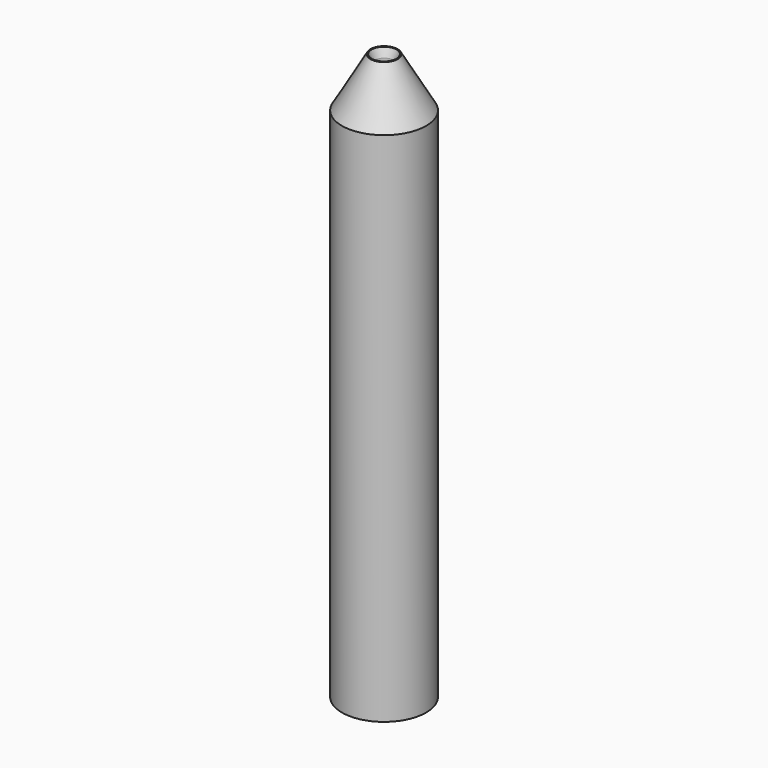
from build123d import *

# Parameters (mm, degrees)
F0_R      = 3.5
F1_DEPTH  = 25
F2_DEPTH  = 47
F3_R      = 1.65
F4_DEPTH  = 38
F5_R      = 1.13
F6_DEPTH  = 100
F6_TAPER  = -30
F8_R      = 1.03
F9_DEPTH  = 2
F9_TAPER  = 22.5
F10_R     = 0.75
F11_DEPTH = 5


# Not quite as in the source:
# - a feature names something its author has since deleted; it is built from what else it names


with BuildPart() as f1:
    # F0 (on Top) → F1 (new body)
    with BuildSketch(Plane.XY):
        Circle(F0_R)
    extrude(amount=F1_DEPTH)


with BuildPart() as f2:
    # F0 (on Top) → F2 (new body)
    with BuildSketch(Plane.XY):
        Circle(F0_R)
    extrude(amount=F2_DEPTH)


with BuildPart() as f4_tool:
    # F3 (on face) → F4 (new body)
    with BuildSketch(Plane(origin=(0, 0, 0), x_dir=(1, 0, 0), z_dir=(0, 0, -1))):
        Circle(F3_R)
    extrude(amount=-F4_DEPTH)


with BuildPart() as f1_1:
    add(f1.part)

    # F4: cut by f4_tool
    add(f4_tool.part, mode=Mode.SUBTRACT)


with BuildPart() as f2_1:
    add(f2.part)

    # F4: cut by f4_tool
    add(f4_tool.part, mode=Mode.SUBTRACT)


with BuildPart() as f6_tool:
    # F5 (on face) → F6 (new body)
    with BuildSketch(Plane.XY.offset(47)):
        Circle(F5_R)
    extrude(amount=-F6_DEPTH, taper=F6_TAPER)


with BuildPart() as f1_2:
    add(f1_1.part)

    # F6: intersect by f6_tool
    add(f6_tool.part, mode=Mode.INTERSECT)


with BuildPart() as f2_2:
    add(f2_1.part)

    # F6: intersect by f6_tool
    add(f6_tool.part, mode=Mode.INTERSECT)

    # F8 (on face) → F9 (cut)
    with BuildSketch(Plane.XY.offset(47)):
        Circle(F8_R)
    extrude(amount=-F9_DEPTH, taper=F9_TAPER, mode=Mode.SUBTRACT)

    # F10 (on face) → F11 (cut)
    with BuildSketch(Plane.XY.offset(47)):
        Circle(F10_R)
    extrude(amount=-F11_DEPTH, mode=Mode.SUBTRACT)


solid = f2_2.part
